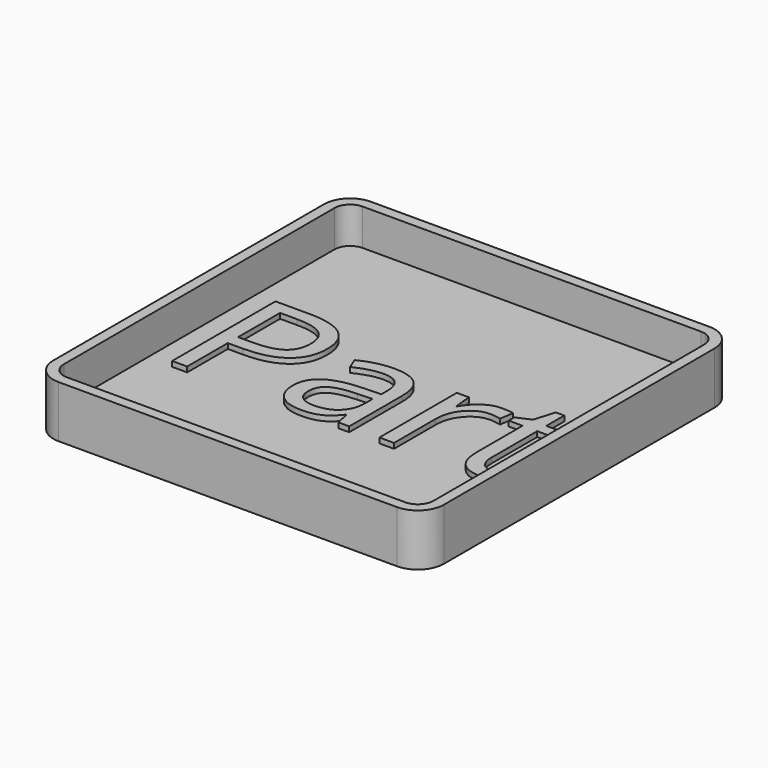
from build123d import *

# Parameters (mm, degrees)
F1_DEPTH     = 3
F2_DEPTH     = 10
F0_TEXT_SIZE = 34.7222222222
F3_DEPTH     = 4


# Not quite as in the source:
# - Text() gives the source's letters only with a copy of the font that has no kerning and outlines rounded to 1/6400 em; it was checked with that copy


with BuildPart() as f1:
    # F0 (on Top) → F1 (new body)
    with BuildSketch(Plane.XY):
        with BuildLine():
            ThreePointArc((-44.6118305922, 5), (-43.7331509357, 2.8786796564), (-41.6118305922, 2))
            Line((-41.6118305922, 2), (23.3881694078, 2))
            ThreePointArc((23.3881694078, 2), (25.5094897514, 2.8786796564), (26.3881694078, 5))
            Line((26.3881694078, 5), (26.3881694078, 70))
            ThreePointArc((26.3881694078, 70), (25.5094897514, 72.1213203436), (23.3881694078, 73))
            Line((23.3881694078, 73), (-41.6118305922, 73))
            ThreePointArc((-41.6118305922, 73), (-43.7331509357, 72.1213203436), (-44.6118305922, 70))
            Line((-44.6118305922, 70), (-44.6118305922, 5))
        make_face()
        with BuildLine():
            add(Edge.make_bspline(
                [(-33.3604200019, 49.7884114583), (-24.0722255574, 49.7884114583), (-24.0722255574, 42.5672743056)],
                knots=[0, 0, 0, 1, 1, 1], degree=2))
            add(Edge.make_bspline(
                [(-24.0722255574, 42.5672743056), (-24.0722255574, 38.8020833333), (-26.6411274672, 36.7757161458)],
                knots=[0, 0, 0, 1, 1, 1], degree=2))
            add(Edge.make_bspline(
                [(-26.6411274672, 36.7757161458), (-29.2100293769, 34.7493489583), (-33.9897602797, 34.7493489583)],
                knots=[0, 0, 0, 1, 1, 1], degree=2))
            Line((-33.9897602797, 34.7493489583), (-36.9085970852, 34.7493489583))
            Line((-36.9085970852, 34.7493489583), (-36.9085970852, 25))
            Line((-36.9085970852, 25), (-39.7894564602, 25))
            Line((-39.7894564602, 25), (-39.7894564602, 49.7884114583))
            Line((-39.7894564602, 49.7884114583), (-33.3604200019, 49.7884114583))
        make_face(mode=Mode.SUBTRACT)
        with BuildLine():
            Line((-5.7942307658, 25), (-7.8829894463, 25))
            Line((-7.8829894463, 25), (-8.4418002102, 27.6475694444))
            Line((-8.4418002102, 27.6475694444), (-8.5774338908, 27.6475694444))
            add(Edge.make_bspline(
                [(-8.5774338908, 27.6475694444), (-9.9663227797, 25.9006076389), (-11.3470736477, 25.2794053819)],
                knots=[0, 0, 0, 1, 1, 1], degree=2))
            add(Edge.make_bspline(
                [(-11.3470736477, 25.2794053819), (-12.7278245158, 24.658203125), (-14.8003071547, 24.658203125)],
                knots=[0, 0, 0, 1, 1, 1], degree=2))
            add(Edge.make_bspline(
                [(-14.8003071547, 24.658203125), (-17.5618088908, 24.658203125), (-19.129734238, 26.0850694444)],
                knots=[0, 0, 0, 1, 1, 1], degree=2))
            add(Edge.make_bspline(
                [(-19.129734238, 26.0850694444), (-20.6976595852, 27.5119357639), (-20.6976595852, 30.1378038194)],
                knots=[0, 0, 0, 1, 1, 1], degree=2))
            add(Edge.make_bspline(
                [(-20.6976595852, 30.1378038194), (-20.6976595852, 35.7638888889), (-11.6970085435, 36.03515625)],
                knots=[0, 0, 0, 1, 1, 1], degree=2))
            Line((-11.6970085435, 36.03515625), (-8.5448818074, 36.1382378472))
            Line((-8.5448818074, 36.1382378472), (-8.5448818074, 37.2938368056))
            add(Edge.make_bspline(
                [(-8.5448818074, 37.2938368056), (-8.5448818074, 39.4802517361), (-9.4834668769, 40.5219184028)],
                knots=[0, 0, 0, 1, 1, 1], degree=2))
            add(Edge.make_bspline(
                [(-9.4834668769, 40.5219184028), (-10.4220519463, 41.5635850694), (-12.4945345852, 41.5635850694)],
                knots=[0, 0, 0, 1, 1, 1], degree=2))
            add(Edge.make_bspline(
                [(-12.4945345852, 41.5635850694), (-14.8165831963, 41.5635850694), (-17.7462706963, 40.1421440972)],
                knots=[0, 0, 0, 1, 1, 1], degree=2))
            Line((-17.7462706963, 40.1421440972), (-18.6143262519, 42.2960069444))
            add(Edge.make_bspline(
                [(-18.6143262519, 42.2960069444), (-17.2417134047, 43.0392795139), (-15.6059712172, 43.4624565972)],
                knots=[0, 0, 0, 1, 1, 1], degree=2))
            add(Edge.make_bspline(
                [(-15.6059712172, 43.4624565972), (-13.9702290297, 43.8856336806), (-12.3209234741, 43.8856336806)],
                knots=[0, 0, 0, 1, 1, 1], degree=2))
            add(Edge.make_bspline(
                [(-12.3209234741, 43.8856336806), (-9.0006109741, 43.8856336806), (-7.3974208699, 42.4126519097)],
                knots=[0, 0, 0, 1, 1, 1], degree=2))
            add(Edge.make_bspline(
                [(-7.3974208699, 42.4126519097), (-5.7942307658, 40.9396701389), (-5.7942307658, 37.6844618056)],
                knots=[0, 0, 0, 1, 1, 1], degree=2))
            Line((-5.7942307658, 37.6844618056), (-5.7942307658, 25))
        make_face(mode=Mode.SUBTRACT)
        with BuildLine():
            add(Edge.make_bspline(
                [(5.2734775676, 42.9389105903), (6.7328959703, 43.9236111111), (8.4798577759, 43.9236111111)],
                knots=[0, 0, 0, 1, 1, 1], degree=2))
            add(Edge.make_bspline(
                [(8.4798577759, 43.9236111111), (9.7168369426, 43.9236111111), (10.6988247898, 43.7174479167)],
                knots=[0, 0, 0, 1, 1, 1], degree=2))
            Line((10.6988247898, 43.7174479167), (10.3081997898, 41.1078559028))
            add(Edge.make_bspline(
                [(10.3081997898, 41.1078559028), (9.1580261787, 41.3628472222), (8.2736945815, 41.3628472222)],
                knots=[0, 0, 0, 1, 1, 1], degree=2))
            add(Edge.make_bspline(
                [(8.2736945815, 41.3628472222), (6.016750137, 41.3628472222), (4.4162727065, 39.5317925347)],
                knots=[0, 0, 0, 1, 1, 1], degree=2))
            add(Edge.make_bspline(
                [(4.4162727065, 39.5317925347), (2.8157952759, 37.7007378472), (2.8157952759, 34.9717881944)],
                knots=[0, 0, 0, 1, 1, 1], degree=2))
            Line((2.8157952759, 34.9717881944), (2.8157952759, 25))
            Line((2.8157952759, 25), (4.00676e-05, 25))
            Line((4.00676e-05, 25), (4.00676e-05, 43.5818142361))
            Line((4.00676e-05, 43.5818142361), (2.3220886787, 43.5818142361))
            Line((2.3220886787, 43.5818142361), (2.647609512, 40.1421440972))
            Line((2.647609512, 40.1421440972), (2.7832431926, 40.1421440972))
            add(Edge.make_bspline(
                [(2.7832431926, 40.1421440972), (3.8140591648, 41.9542100694), (5.2734775676, 42.9389105903)],
                knots=[0, 0, 0, 1, 1, 1], degree=2))
        make_face(mode=Mode.SUBTRACT)
        with BuildLine():
            add(Edge.make_bspline(
                [(17.9904914565, 27.8835720486), (18.7880174981, 26.9856770833), (20.176906387, 26.9856770833)],
                knots=[0, 0, 0, 1, 1, 1], degree=2))
            add(Edge.make_bspline(
                [(20.176906387, 26.9856770833), (20.9256043037, 26.9856770833), (21.6200487481, 27.0941840278)],
                knots=[0, 0, 0, 1, 1, 1], degree=2))
            add(Edge.make_bspline(
                [(21.6200487481, 27.0941840278), (22.3144931926, 27.2026909722), (22.7213942342, 27.3220486111)],
                knots=[0, 0, 0, 1, 1, 1], degree=2))
            Line((22.7213942342, 27.3220486111), (22.7213942342, 25.1681857639))
            add(Edge.make_bspline(
                [(22.7213942342, 25.1681857639), (22.2656650676, 24.951171875), (21.3759081231, 24.8046875)],
                knots=[0, 0, 0, 1, 1, 1], degree=2))
            add(Edge.make_bspline(
                [(21.3759081231, 24.8046875), (20.4861511787, 24.658203125), (19.7700053453, 24.658203125)],
                knots=[0, 0, 0, 1, 1, 1], degree=2))
            add(Edge.make_bspline(
                [(19.7700053453, 24.658203125), (14.3826355537, 24.658203125), (14.3826355537, 30.3385416667)],
                knots=[0, 0, 0, 1, 1, 1], degree=2))
            Line((14.3826355537, 30.3385416667), (14.3826355537, 41.3953993056))
            Line((14.3826355537, 41.3953993056), (11.7187900676, 41.3953993056))
            Line((11.7187900676, 41.3953993056), (11.7187900676, 42.7517361111))
            Line((11.7187900676, 42.7517361111), (14.3826355537, 43.9236111111))
            Line((14.3826355537, 43.9236111111), (15.5653612481, 47.8895399306))
            Line((15.5653612481, 47.8895399306), (17.1929654148, 47.8895399306))
            Line((17.1929654148, 47.8895399306), (17.1929654148, 43.5818142361))
            Line((17.1929654148, 43.5818142361), (22.5857605537, 43.5818142361))
            Line((22.5857605537, 43.5818142361), (22.5857605537, 41.3953993056))
            Line((22.5857605537, 41.3953993056), (17.1929654148, 41.3953993056))
            Line((17.1929654148, 41.3953993056), (17.1929654148, 30.4578993056))
            add(Edge.make_bspline(
                [(17.1929654148, 30.4578993056), (17.1929654148, 28.7814670139), (17.9904914565, 27.8835720486)],
                knots=[0, 0, 0, 1, 1, 1], degree=2))
        make_face(mode=Mode.SUBTRACT)
    extrude(amount=F1_DEPTH)

    # F0 (on Top) → F2 (join)
    with BuildSketch(Plane.XY):
        with BuildLine():
            Line((23.3881694078, 75), (-41.6118305922, 75))
            ThreePointArc((-41.6118305922, 75), (-45.1473644981, 73.5355339059), (-46.6118305922, 70))
            Line((-46.6118305922, 70), (-46.6118305922, 5))
            ThreePointArc((-46.6118305922, 5), (-45.1473644981, 1.4644660941), (-41.6118305922, 0))
            Line((-41.6118305922, 0), (23.3881694078, 0))
            ThreePointArc((23.3881694078, 0), (26.9237033138, 1.4644660941), (28.3881694078, 5))
            Line((28.3881694078, 5), (28.3881694078, 70))
            ThreePointArc((28.3881694078, 70), (26.9237033138, 73.5355339059), (23.3881694078, 75))
        make_face()
        with BuildLine():
            Line((23.3881694078, 2), (-41.6118305922, 2))
            ThreePointArc((-41.6118305922, 2), (-43.7331509357, 2.8786796564), (-44.6118305922, 5))
            Line((-44.6118305922, 5), (-44.6118305922, 70))
            ThreePointArc((-44.6118305922, 70), (-43.7331509357, 72.1213203436), (-41.6118305922, 73))
            Line((-41.6118305922, 73), (23.3881694078, 73))
            ThreePointArc((23.3881694078, 73), (25.5094897514, 72.1213203436), (26.3881694078, 70))
            Line((26.3881694078, 70), (26.3881694078, 5))
            ThreePointArc((26.3881694078, 5), (25.5094897514, 2.8786796564), (23.3881694078, 2))
        make_face(mode=Mode.SUBTRACT)
    extrude(amount=F2_DEPTH)



with BuildPart() as f1b:
    # F0 (on Top) → F1, piece 2 (new body)
    with BuildSketch(Plane.XY):
        with BuildLine():
            add(Edge.make_bspline(
                [(-16.8239616685, 27.7804904514), (-15.9016526408, 26.9856770833), (-14.2414963908, 26.9856770833)],
                knots=[0, 0, 0, 1, 1, 1], degree=2))
            add(Edge.make_bspline(
                [(-14.2414963908, 26.9856770833), (-11.610202988, 26.9856770833), (-10.110094481, 28.4261067708)],
                knots=[0, 0, 0, 1, 1, 1], degree=2))
            add(Edge.make_bspline(
                [(-10.110094481, 28.4261067708), (-8.6099859741, 29.8665364583), (-8.6099859741, 32.4598524306)],
                knots=[0, 0, 0, 1, 1, 1], degree=2))
            Line((-8.6099859741, 32.4598524306), (-8.6099859741, 34.1362847222))
            Line((-8.6099859741, 34.1362847222), (-11.4257411824, 34.0223524306))
            add(Edge.make_bspline(
                [(-11.4257411824, 34.0223524306), (-14.784031113, 33.9029947917), (-16.2651509047, 32.9779730903)],
                knots=[0, 0, 0, 1, 1, 1], degree=2))
            add(Edge.make_bspline(
                [(-16.2651509047, 32.9779730903), (-17.7462706963, 32.0529513889), (-17.7462706963, 30.1052517361)],
                knots=[0, 0, 0, 1, 1, 1], degree=2))
            add(Edge.make_bspline(
                [(-17.7462706963, 30.1052517361), (-17.7462706963, 28.5753038194), (-16.8239616685, 27.7804904514)],
                knots=[0, 0, 0, 1, 1, 1], degree=2))
        make_face()
    extrude(amount=F1_DEPTH)


with BuildPart() as f1c:
    # F0 (on Top) → F1, piece 3 (new body)
    with BuildSketch(Plane.XY):
        with BuildLine():
            Line((-36.9085970852, 47.2927517361), (-36.9085970852, 37.2233072917))
            Line((-36.9085970852, 37.2233072917), (-34.3098557658, 37.2233072917))
            add(Edge.make_bspline(
                [(-34.3098557658, 37.2233072917), (-30.4795606269, 37.2233072917), (-28.7678635783, 38.4602864583)],
                knots=[0, 0, 0, 1, 1, 1], degree=2))
            add(Edge.make_bspline(
                [(-28.7678635783, 38.4602864583), (-27.0561665297, 39.697265625), (-27.0561665297, 42.431640625)],
                knots=[0, 0, 0, 1, 1, 1], degree=2))
            add(Edge.make_bspline(
                [(-27.0561665297, 42.431640625), (-27.0561665297, 44.8893229167), (-28.6674946547, 46.0910373264)],
                knots=[0, 0, 0, 1, 1, 1], degree=2))
            add(Edge.make_bspline(
                [(-28.6674946547, 46.0910373264), (-30.2788227797, 47.2927517361), (-33.6859408352, 47.2927517361)],
                knots=[0, 0, 0, 1, 1, 1], degree=2))
            Line((-33.6859408352, 47.2927517361), (-36.9085970852, 47.2927517361))
        make_face()
    extrude(amount=F1_DEPTH)


with BuildPart() as f1_1:
    add(f1.part)

    add(f1b.part)  # F3 merges F1b

    add(f1c.part)  # F3 merges F1c
    # F0 (on Top) → F3 (join)
    with BuildSketch(Plane.XY):
        with Locations((-43.1965745158, 25)):
            Text('Part', F0_TEXT_SIZE, font='Open Sans', text_align=(TextAlign.LEFT, TextAlign.BOTTOM))
    extrude(amount=F3_DEPTH)


solid = f1_1.part
